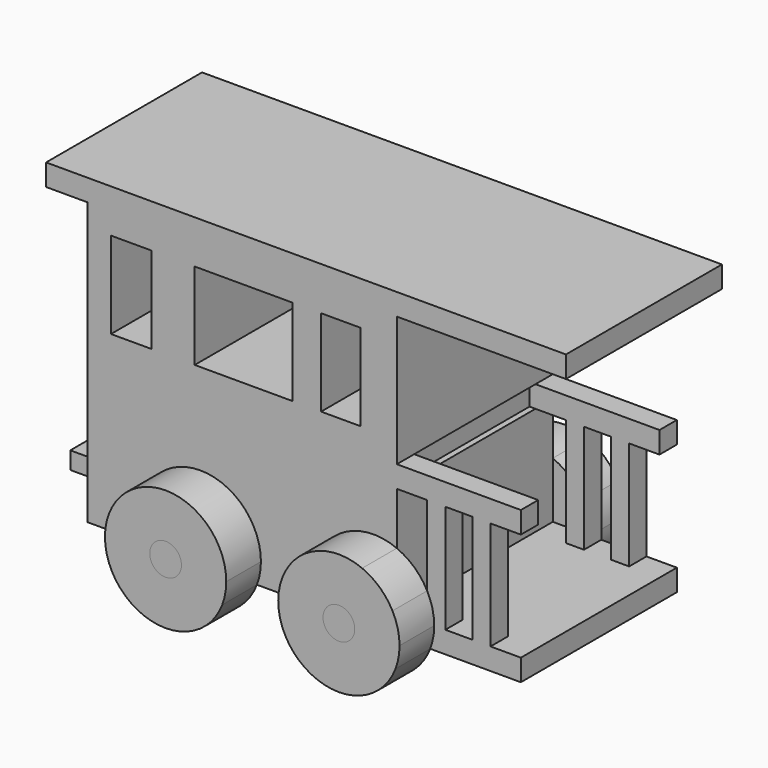
from build123d import *

# Parameters (mm, degrees)
F0_W           = 5.334
F0_H           = 31.75
F0_W_2         = 12.1767708808
F0_H_2         = 6.35
F0_W_3         = 13.2232291192
F0_W_4         = 11.8282231389
F0_H_3         = 25.4
F0_W_5         = 28.695857618
F0_W_6         = 11.6236433387
F1_DEPTH       = 28.575
F2_W           = 44.45
F2_H           = 31.75
F3_DEPTH       = 25.4
F4_W           = 44.45
F4_H           = 6.35
F5_DEPTH       = 38.1
F6_R           = 4.6482
F7_DEPTH       = 12.7
F9_DEPTH       = 12.7
F9_DEPTH_BACK  = 70.104
F10_W          = 25.4
F10_H          = 5.08
F11_DEPTH      = 17.78
F12_R          = 6.35
F13_DEPTH      = 17.78
F14_DEPTH      = 69.85
F14_DEPTH_BACK = 12.7


# Not quite as in the source:
# - a feature names something its author has since deleted; it is built from what else it names


with BuildPart() as f1:
    # F0 (on Front) → F1 (new body, symmetric)
    with BuildSketch(Plane.XZ):
        Polygon((40.5938484461, 0), (35.2598484461, 0), (35.2598484461, -20.7330111994), (35.2598484461, -31.75), (40.5938484461, -31.75), (40.5938484461, -22.8515356839), align=None)
        with Locations((51.1692069136, -15.875)):
            Rectangle(F0_W, F0_H)
        with Locations((-70.3621785268, 47.625)):
            Rectangle(F0_W_2, F0_H_2)
        with Locations((69.3378214732, 47.625)):
            Rectangle(F0_W_3, F0_H_2)
        Polygon((62.7262069136, 50.8), (-64.2737930864, 50.8), (-64.2737930864, 44.45), (26.3698484461, 44.45), (62.7262069136, 44.45), align=None)
        Polygon((26.3698484461, 44.45), (-64.2737930864, 44.45), (-64.2737930864, -38.1), (-47.8611980613, -38.1), (-14.6463881115, -38.1), (13.0988019387, -38.1), (26.3698484461, -38.1), (26.3698484461, -31.75), (26.3698484461, -14.7111620115), (26.3698484461, 0), (26.3698484461, 6.35), align=None)
        with Locations((-51.5087349863, 25.4)):
            Rectangle(F0_W_4, F0_H_3, mode=Mode.SUBTRACT)
        with Locations((-18.5333405269, 25.4)):
            Rectangle(F0_W_5, F0_H_3, mode=Mode.SUBTRACT)
        with Locations((9.980898246, 25.4)):
            Rectangle(F0_W_6, F0_H_3, mode=Mode.SUBTRACT)
        Polygon((62.7262069136, 0), (62.7262069136, 6.35), (26.3698484461, 6.35), (26.3698484461, 0), (35.2598484461, 0), (40.5938484461, 0), (48.5022069136, 0), (53.8362069136, 0), align=None)
        Polygon((62.7262069136, -38.1), (62.7262069136, -31.75), (53.8362069136, -31.75), (48.5022069136, -31.75), (47.4862069136, -31.75), (40.5938484461, -31.75), (35.2598484461, -31.75), (26.3698484461, -31.75), (26.3698484461, -38.1), (46.3136118885, -38.1), align=None)
    extrude(amount=F1_DEPTH, both=True)

    # F2 (on face) → F3 (cut)
    with BuildSketch(Plane.YZ.offset(53.8362069136)):
        with Locations((0, -15.875)):
            Rectangle(F2_W, F2_H)
    extrude(amount=-F3_DEPTH, mode=Mode.SUBTRACT)

    # F4 (on face) → F5 (cut)
    with BuildSketch(Plane.YZ.offset(62.7262069136)):
        with Locations((0, 3.175)):
            Rectangle(F4_W, F4_H)
    extrude(amount=-F5_DEPTH, mode=Mode.SUBTRACT)

    # F6 (on face) → F9 (cut, two sides)
    with BuildSketch(Plane.XZ.offset(28.575)) as f9_sk:
        with Locations((19.5462069136, -31.75)):
            Circle(F6_R)
        with Locations((-31.2537930864, -31.75)):
            Circle(F6_R)
    extrude(amount=F9_DEPTH, mode=Mode.SUBTRACT)
    extrude(f9_sk.sketch, amount=-F9_DEPTH_BACK, mode=Mode.SUBTRACT)

    # F10 (on face) → F11 (join)
    with BuildSketch(Plane(origin=(-64.2737930864, 0, 0), x_dir=(0, -1, 0), z_dir=(-1, 0, 0))):
        with Locations((0, -34.3196164)):
            Rectangle(F10_W, F10_H)
    extrude(amount=F11_DEPTH)

    # F12 (on face) → F13 (join)
    with BuildSketch(Plane.XY.offset(-31.7796164)):
        with Locations((-73.6990726864, 0)):
            Circle(F12_R)
    extrude(amount=F13_DEPTH)


with BuildPart() as f7:
    # F6 (on face) → F7 (new body)
    with BuildSketch(Plane.XZ.offset(28.575)):
        with BuildLine():
            ThreePointArc((36.1536118885, -38.1), (37.0306008186, -34.9786792614), (37.3262069136, -31.75))
            ThreePointArc((37.3262069136, -31.75), (36.8018863619, -27.4639847439), (35.2598484461, -23.4307530517))
            Line((35.2598484461, -23.4307530517), (35.2598484461, -31.75))
            Line((35.2598484461, -31.75), (26.3698484461, -31.75))
            Line((26.3698484461, -31.75), (26.3698484461, -15.331525155))
            ThreePointArc((26.3698484461, -15.331525155), (7.1554293566, -18.9986458941), (2.9388019387, -38.1))
            Line((2.9388019387, -38.1), (36.1536118885, -38.1))
        make_face()
        with Locations((19.5462069136, -31.75)):
            Circle(F6_R, mode=Mode.SUBTRACT)
        with BuildLine():
            Line((35.2598484461, -31.75), (35.2598484461, -23.4307530517))
            ThreePointArc((35.2598484461, -23.4307530517), (31.5204148256, -18.6066844031), (26.3698484461, -15.331525155))
            Line((26.3698484461, -15.331525155), (26.3698484461, -31.75))
            Line((26.3698484461, -31.75), (35.2598484461, -31.75))
        make_face()
        with BuildLine():
            ThreePointArc((2.9388019387, -38.1), (19.5462069136, -49.53), (36.1536118885, -38.1))
            Line((36.1536118885, -38.1), (2.9388019387, -38.1))
        make_face()
    extrude(amount=F7_DEPTH)


with BuildPart() as f7b:
    # F6 (on face) → F7, piece 2 (new body)
    with BuildSketch(Plane.XZ.offset(28.575)):
        with BuildLine():
            Line((-47.8611980613, -38.1), (-14.6463881115, -38.1))
            ThreePointArc((-14.6463881115, -38.1), (-13.7693991814, -34.9786792614), (-13.4737930864, -31.75))
            ThreePointArc((-13.4737930864, -31.75), (-34.4824723478, -14.265606095), (-47.8611980613, -38.1))
        make_face()
        with Locations((-31.2537930864, -31.75)):
            Circle(F6_R, mode=Mode.SUBTRACT)
        with BuildLine():
            ThreePointArc((-47.8611980613, -38.1), (-31.2537930864, -49.53), (-14.6463881115, -38.1))
            Line((-14.6463881115, -38.1), (-47.8611980613, -38.1))
        make_face()
    extrude(amount=F7_DEPTH)


with BuildPart() as f8_1:
    # F8: instance of F7
    add(f7.part.mirror(Plane.XZ))


with BuildPart() as f8_2:
    # F8: instance of F7b
    add(f7b.part.mirror(Plane.XZ))


with BuildPart() as f14:
    # F6 (on face) → F14 (new body, two sides)
    with BuildSketch(Plane.XZ.offset(28.575)) as f14_sk:
        with Locations((-31.2537930864, -31.75)):
            Circle(F6_R)
    extrude(amount=-F14_DEPTH)
    extrude(f14_sk.sketch, amount=F14_DEPTH_BACK)


with BuildPart() as f14b:
    # F6 (on face) → F14, piece 2 (new body, two sides)
    with BuildSketch(Plane.XZ.offset(28.575)) as f14_2_sk:
        with Locations((19.5462069136, -31.75)):
            Circle(F6_R)
    extrude(amount=-F14_DEPTH)
    extrude(f14_2_sk.sketch, amount=F14_DEPTH_BACK)


solid = Compound([f1.part, f7.part, f7b.part, f8_1.part, f8_2.part, f14.part, f14b.part])
